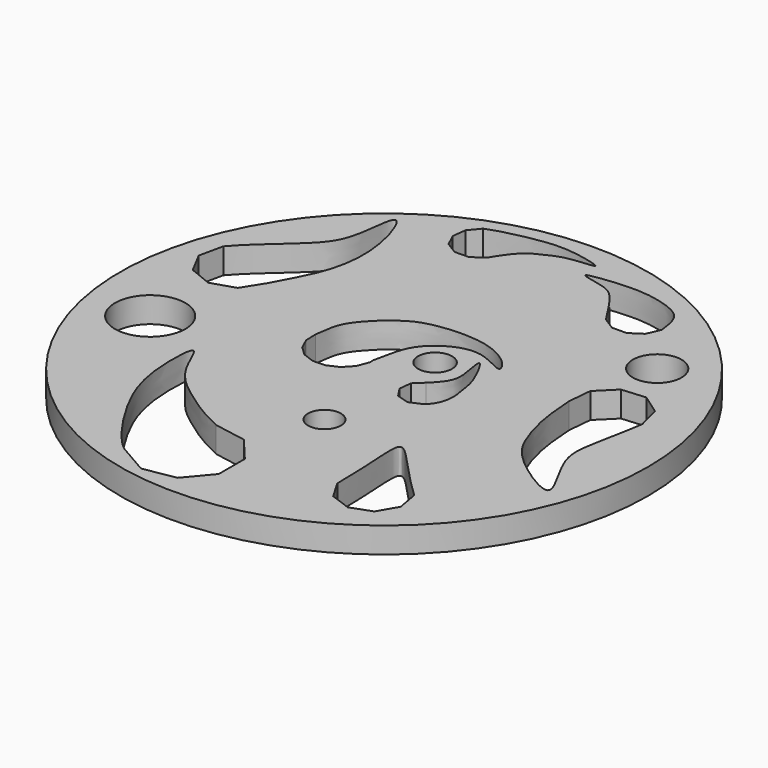
from build123d import *

# Parameters (mm, degrees)
F0_R     = 31
F0_R_2   = 4.1365832931
F0_R_3   = 1.9275687043
F0_R_4   = 2.0005563938
F0_R_5   = 2.8578450459
F1_DEPTH = 3


with BuildPart() as f1:
    # F0 (on Top) → F1 (new body)
    with BuildSketch(Plane.XY):
        with Locations((0.1946801621, 0.3926200628)):
            Circle(F0_R)
        with BuildLine():
            Line((-1.1422014806, -18.5189035409), (1.3240849968, -21.4581093107))
            Line((1.3240849968, -21.4581093107), (1.3240849968, -25.2949699475))
            Line((1.3240849968, -25.2949699475), (-1.1422014806, -28.2341757172))
            Line((-1.1422014806, -28.2341757172), (-4.9207715829, -28.9004395748))
            Line((-4.9207715829, -28.9004395748), (-8.5211597808, -26.8217544795))
            add(Edge.make_bspline(
                [(-4.9207715829, -17.8526396834), (-6.9909564865, -16.9647118268), (-10.7168431989, -14.4933921603), (-14.1859433865, -11.5381742982), (-16.131211939, -5.6113285497), (-16.3999346819, -12.6545592251), (-15.0544363476, -17.8264461458), (-11.732939874, -23.3115263439), (-9.6781806545, -25.9427554538), (-8.5211597808, -26.8217544795)],
                knots=[0, 0, 0, 0, 0.1618028325, 0.3035028648, 0.4217425117, 0.5509588088, 0.7069372822, 0.8641646726, 1, 1, 1, 1], degree=3))
            Line((-4.9207715829, -17.8526396834), (-1.1422014806, -18.5189035409))
        make_face(mode=Mode.SUBTRACT)
        with Locations((-23.1914689183, -4.7165894897)):
            Circle(F0_R_2, mode=Mode.SUBTRACT)
        with BuildLine():
            add(Edge.make_bspline(
                [(10.9767442969, -19.9434975307), (10.9767442969, -14.2306106595), (9.5908596585, -7.470016463), (13.8118869508, -13.4848055604), (17.9670492103, -17.3992346138)],
                knots=[0, 0, 0, 0, 0.4943486381, 1, 1, 1, 1], degree=3))
            Line((17.9670492103, -17.3992346138), (18.4156714086, -19.9434975307))
            Line((18.4156714086, -19.9434975307), (17.1239152718, -22.1808847906))
            Line((17.1239152718, -22.1808847906), (14.6962078527, -23.0644980286))
            Line((14.6962078527, -23.0644980286), (12.2685004336, -22.1808847906))
            Line((12.2685004336, -22.1808847906), (10.9767442969, -19.9434975307))
        make_face(mode=Mode.SUBTRACT)
        with Locations((2.1389996326, -10.7908323988)):
            Circle(F0_R_3, mode=Mode.SUBTRACT)
        with BuildLine():
            add(Edge.make_bspline(
                [(17.3791687237, 6.0507453724), (17.4829293163, 4.6126524003), (17.6881609354, 1.7868632521), (18.8410094769, -2.1760334773), (20.5826203099, -5.6656983025), (29.3238900367, -11.300011281), (24.1806930972, -3.7954405403), (24.0697865205, -0.71520103), (24.7682450981, 2.7334855195), (25.2540633757, 5.1594822195), (25.4738810638, 6.724710861)],
                knots=[0, 0, 0, 0, 0.1239250683, 0.2415906445, 0.3695409376, 0.5199879999, 0.6573859161, 0.7702265486, 0.877856999, 1, 1, 1, 1], degree=3))
            Line((17.3791687237, 6.0507453724), (17.6368298374, 8.8599451395))
            Line((17.6368298374, 8.8599451395), (19.6399285052, 10.8462956392))
            Line((19.6399285052, 10.8462956392), (22.4511925984, 11.080361397))
            Line((22.4511925984, 11.080361397), (24.7552004041, 9.4526204434))
            Line((24.7552004041, 9.4526204434), (25.4738810638, 6.724710861))
        make_face(mode=Mode.SUBTRACT)
        with BuildLine():
            add(Edge.make_bspline(
                [(-18.8531623265, 7.1124824437), (-18.0146350035, 8.8593640986), (-15.8735436071, 12.0524492088), (-14.9743904527, 18.9530716251), (-17.9386034601, 26.6079568134), (-18.2197344554, 19.4240488252), (-20.0397954496, 15.9479840875), (-24.5950836461, 12.5983474658), (-26.5965992132, 10.2770576194)],
                knots=[0, 0, 0, 0, 0.1648856245, 0.3554270756, 0.5091783331, 0.6514727109, 0.7966248505, 1, 1, 1, 1], degree=3))
            Line((-18.8531623265, 7.1124824437), (-20.4024971664, 4.6549182851))
            Line((-20.4024971664, 4.6549182851), (-23.1690483022, 3.7682081561))
            Line((-23.1690483022, 3.7682081561), (-25.8583157107, 4.8672535807))
            Line((-25.8583157107, 4.8672535807), (-27.2119612836, 7.4377989904))
            Line((-27.2119612836, 7.4377989904), (-26.5965992132, 10.2770576194))
        make_face(mode=Mode.SUBTRACT)
        with BuildLine():
            add(Edge.make_bspline(
                [(-1.7272980043, 1.2194981841), (-1.7219491873, 1.0434659123), (-1.7166003704, 0.8674336406), (-1.7112515534, 0.6914013688)],
                knots=[0, 0, 0, 0, 0.5283405483, 0.5283405483, 0.5283405483, 0.5283405483], degree=3))
            Line((-1.7112515534, 0.6914013688), (-2.2266321603, -0.6682363927))
            Line((-2.2266321603, -0.6682363927), (-3.2230925997, -1.7271502725))
            Line((-3.2230925997, -1.7271502725), (-4.5489308027, -2.3241302316))
            Line((-4.5489308027, -2.3241302316), (-6.0022999218, -2.3682914828))
            Line((-6.0022999218, -2.3682914828), (-7.3619376832, -1.852910876))
            Line((-7.3619376832, -1.852910876), (-8.420851563, -0.8564504365))
            Line((-8.420851563, -0.8564504365), (-9.0178315221, 0.4693877665))
            Line((-9.0178315221, 0.4693877665), (-9.0619927733, 1.9227568855))
            add(Edge.make_bspline(
                [(-9.0619927733, 1.9227568855), (-8.8179008554, 3.564503481), (-8.7368035813, 5.3092127127), (-4.7663528657, 9.2209920717), (-1.4153652629, 10.4004575787), (4.5563847989, 10.6369311157), (8.0782344465, 8.3127273723), (8.747287529, 6.4305452611), (5.3022202088, 8.8766445635), (1.7841099871, 7.8708167043), (-0.630612326, 5.7339658841), (-1.3795391649, 3.0876786056), (-1.5027476697, 2.0934057257), (-1.7272980043, 1.2194981841)],
                knots=[0, 0, 0, 0, 0.0949582783, 0.206551198, 0.3033765102, 0.4253453535, 0.5279971179, 0.5747596359, 0.6626653595, 0.7594766074, 0.8485909582, 0.9281812992, 0.9993665584, 0.9993665584, 0.9993665584, 0.9993665584], degree=3))
        make_face(mode=Mode.SUBTRACT)
        with BuildLine():
            add(Edge.make_bspline(
                [(-10.1829958127, 27.9149531313), (-9.2147696429, 28.3094194496), (-7.0695223864, 28.8705887737), (-3.2908756665, 29.6040592936), (-0.2536438221, 29.4256325965), (3.8782219705, 28.3636429154), (-0.6450782687, 28.360332478), (-2.5696827244, 27.2938452286), (-4.3148545094, 26.6240290951), (-5.6371197048, 24.7830766655), (-6.3147368559, 23.5987893069)],
                knots=[0, 0, 0, 0, 0.1323665743, 0.2744295955, 0.4129123579, 0.5261743392, 0.648548582, 0.764675842, 0.8604623277, 1, 1, 1, 1], degree=3))
            Line((-6.3147368559, 23.5987893069), (-7.6874323935, 22.6838097824))
            Line((-7.6874323935, 22.6838097824), (-9.3368926421, 22.6562152625))
            Line((-9.3368926421, 22.6562152625), (-10.7394256273, 23.5247668123))
            Line((-10.7394256273, 23.5247668123), (-11.4497370361, 25.0137054517))
            Line((-11.4497370361, 25.0137054517), (-11.242308015, 26.6503036829))
            Line((-11.242308015, 26.6503036829), (-10.1829958127, 27.9149531313))
        make_face(mode=Mode.SUBTRACT)
        with BuildLine():
            add(Edge.make_bspline(
                [(4.8348368809, 0.7353488595), (5.4489169037, 1.3074735731), (6.748716136, 2.7091540079), (6.4570504869, 4.8212247028), (5.8288014151, 8.024305967), (7.9506600098, 4.0510234784), (8.2348759594, 2.509987015), (8.4334547204, 1.3611032539), (8.7051767486, -0.4608636504), (8.0152749224, -2.1162070331), (7.5015709254, -2.5718468674), (7.2639224009, -2.7444747645)],
                knots=[0, 0, 0, 0, 0.1306935807, 0.2562881533, 0.3636277771, 0.5051531931, 0.6170593609, 0.7022792464, 0.8129661585, 0.9208945849, 1, 1, 1, 1], degree=3))
            Line((7.2639224009, -2.7444747645), (5.9082172801, -3.3367482799))
            Line((5.9082172801, -3.3367482799), (4.4889808287, -2.9190256612))
            Line((4.4889808287, -2.9190256612), (3.6702895552, -1.6867639641))
            Line((3.6702895552, -1.6867639641), (3.8352182052, -0.2165521318))
            Line((3.8352182052, -0.2165521318), (4.8348368809, 0.7353488595))
        make_face(mode=Mode.SUBTRACT)
        with Locations((2.9879567598, 4.3863726313)):
            Circle(F0_R_4, mode=Mode.SUBTRACT)
        with BuildLine():
            Line((14.9090430899, 24.1260071552), (15.1698025284, 22.4394930436))
            Line((15.1698025284, 22.4394930436), (14.4773689593, 20.879729893))
            Line((14.4773689593, 20.879729893), (13.0515851483, 19.941931483))
            Line((13.0515851483, 19.941931483), (11.3451273812, 19.9238421826))
            Line((11.3451273812, 19.9238421826), (9.8997839419, 20.8312052169))
            add(Edge.make_bspline(
                [(9.8997839419, 20.8312052169), (8.9390931135, 22.3405406549), (7.3311606242, 24.8667534764), (5.7755384173, 25.9183575041), (1.3003343599, 26.564740684), (6.7260565905, 27.2369968987), (10.2149852059, 27.2430659991), (14.2375450805, 25.9727334709), (14.7153726717, 24.6586316051), (14.9090430899, 24.1260071552)],
                knots=[0, 0, 0, 0, 0.1754251721, 0.2936135386, 0.4224230604, 0.5678260556, 0.7359203963, 0.8929647257, 1, 1, 1, 1], degree=3))
        make_face(mode=Mode.SUBTRACT)
        with Locations((19.649013007, 16.1707739057)):
            Circle(F0_R_5, mode=Mode.SUBTRACT)
    extrude(amount=F1_DEPTH)


solid = f1.part
